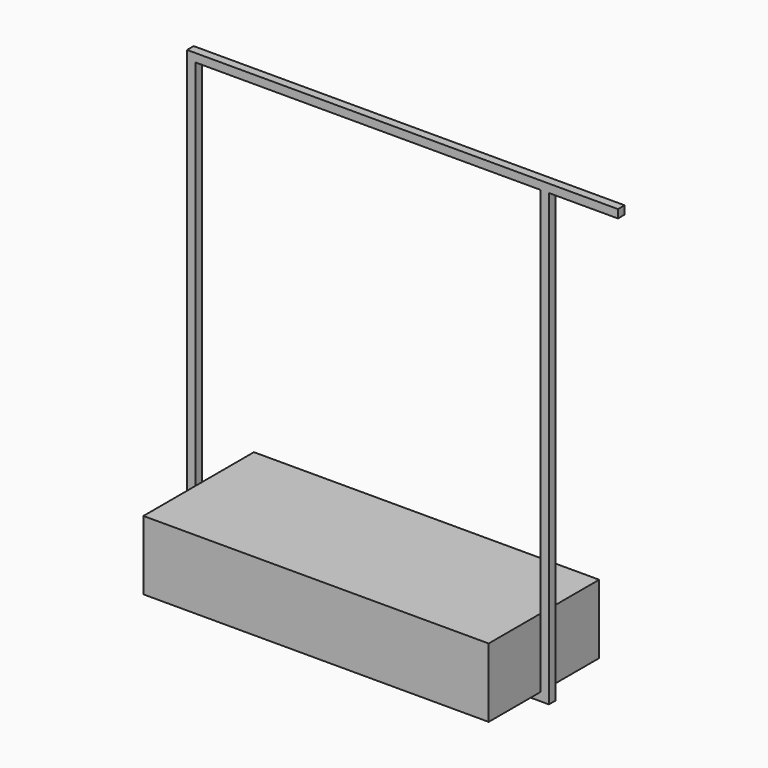
from build123d import *

# Parameters (mm, degrees)
F0_W     = 1250
F0_H     = 500
F1_DEPTH = 250
F2_W     = 1310
F2_H     = 1660
F2_W_2   = 1250
F2_H_2   = 1600
F3_DEPTH = 15
F4_W     = 1050
F4_H     = 300
F4_W_2   = 990
F4_H_2   = 240
F5_DEPTH = 30
F6_W     = 30
F6_H     = 30
F7_DEPTH = 250


with BuildPart() as f1:
    # F0 (on Top) → F1 (new body)
    with BuildSketch(Plane.XY):
        Rectangle(F0_W, F0_H)
    extrude(amount=F1_DEPTH)


with BuildPart() as f3:
    # F2 (on Front) → F3 (new body, symmetric)
    with BuildSketch(Plane.XZ):
        with Locations((0, 800)):
            Rectangle(F2_W, F2_H)
        with Locations((0, 800)):
            Rectangle(F2_W_2, F2_H_2, mode=Mode.SUBTRACT)
    extrude(amount=F3_DEPTH, both=True)

    # F4 (on face) → F5 (join)
    with BuildSketch(Plane(origin=(0, 0, 0), x_dir=(1, 0, 0), z_dir=(0, 0, -1))):
        Rectangle(F4_W, F4_H)
        Rectangle(F4_W_2, F4_H_2, mode=Mode.SUBTRACT)
    extrude(amount=F5_DEPTH)

    # F6 (on face) → F7 (join)
    with BuildSketch(Plane.YZ.offset(655)):
        with Locations((0, 1615)):
            Rectangle(F6_W, F6_H)
    extrude(amount=F7_DEPTH)


solid = Compound([f1.part, f3.part])
